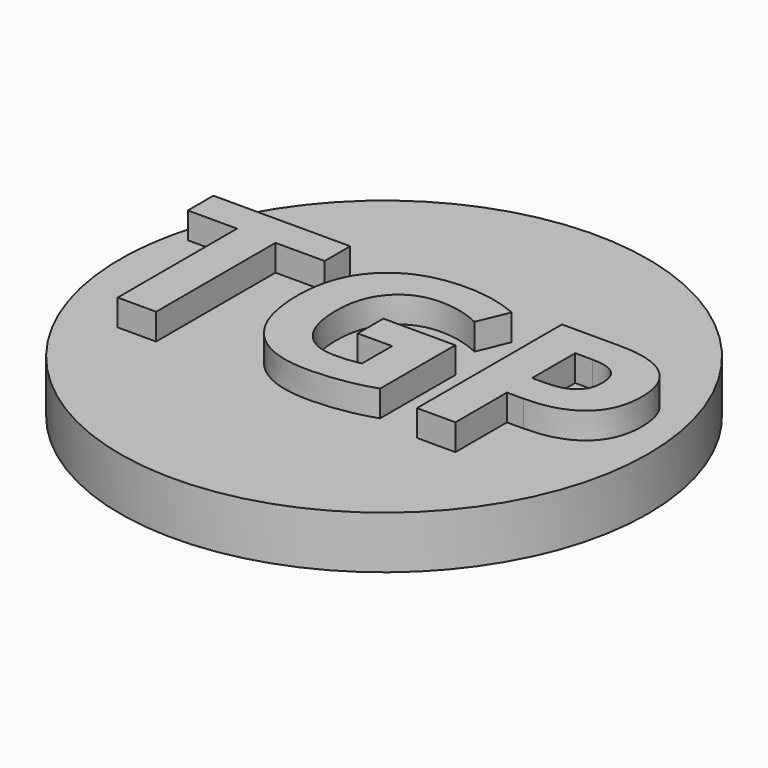
from build123d import *

# Parameters (mm, degrees)
F0_R         = 25.5314110883
F1_DEPTH     = 5.08
F2_TEXT_SIZE = 24.5546639418
F3_DEPTH     = 2.54


# Not quite as in the source:
# - Text() gives the source's letters only with a copy of the font that has no kerning and outlines rounded to 1/6400 em; it was checked with that copy


with BuildPart() as f1:
    # F0 (on Top) → F1 (new body)
    with BuildSketch(Plane.XY):
        Circle(F0_R)
    extrude(amount=F1_DEPTH)

    # F2 (on face) → F3 (join)
    with BuildSketch(Plane.XY.offset(5.08)):
        with Locations((-23.9523073419, -8.839679019)):
            Text('TGP', F2_TEXT_SIZE, font='Open Sans', font_style=FontStyle.BOLD, text_align=(TextAlign.LEFT, TextAlign.BOTTOM))
    extrude(amount=F3_DEPTH)


solid = f1.part
